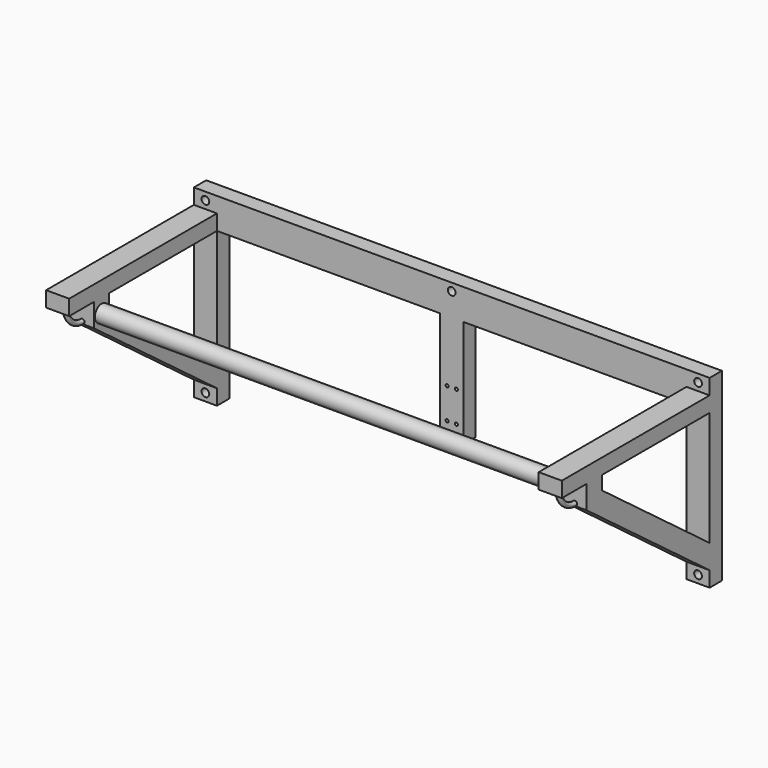
from build123d import *

# Parameters (mm, degrees)
F0_W           = 38.1
F0_H           = 25.4
F0_W_2         = 368.3
F0_H_2         = 177.8
F0_H_3         = 254
F1_DEPTH       = 25.4
F2_W           = 38.1
F2_H           = 25.4
F3_DEPTH       = 304.8
F4_W           = 850.9
F4_H           = 25.4
F5_DEPTH       = 25.4
F7_DEPTH       = 38.1
F9_DEPTH       = 38.1
F10_R          = 2.54
F11_DEPTH      = 12.7
F12_R          = 13.97
F13_DEPTH      = 406.4
F13_DEPTH_BACK = 406.4
F15_DEPTH      = 38.1
F17_DEPTH      = 38.1
F18_W          = 15.24
F18_H          = 39.0179467559
F19_DEPTH      = 50.8
F20_W          = 15.24
F20_H          = 39.0179467559
F21_DEPTH      = 50.8
F22_R          = 3.80999
F23_R          = 3.81
F24_DEPTH      = 25.4
F25_R          = 6.35
F26_DEPTH      = 12.7
F27_R          = 6.35
F28_DEPTH      = 12.7
F29_R          = 6.35
F30_DEPTH      = 12.7


# Not quite as in the source:
# - a fillet or chamfer is up to 0.001 mm smaller than in the source, because OpenCascade refuses the exact size


with BuildPart() as f1:
    # F0 (on Front) → F1 (new body)
    with BuildSketch(Plane.XZ):
        with Locations((0, 139.7)):
            Rectangle(F0_W, F0_H)
        with Locations((203.2, 114.3)):
            Rectangle(F0_W_2, F0_H)
        with Locations((0, 114.3)):
            Rectangle(F0_W, F0_H)
        with Locations((-203.2, 114.3)):
            Rectangle(F0_W_2, F0_H)
        with Locations((0, 12.7)):
            Rectangle(F0_W, F0_H_2)
        with Locations((406.4, 114.3)):
            Rectangle(F0_W, F0_H)
        with Locations((406.4, 139.7)):
            Rectangle(F0_W, F0_H)
        with Locations((-406.4, 139.7)):
            Rectangle(F0_W, F0_H)
        with Locations((-406.4, 114.3)):
            Rectangle(F0_W, F0_H)
        with Locations((406.4, -25.4)):
            Rectangle(F0_W, F0_H_3)
        with Locations((-406.4, -25.4)):
            Rectangle(F0_W, F0_H_3)
    extrude(amount=F1_DEPTH)

    # F2 (on face) → F3 (join)
    with BuildSketch(Plane.XZ.offset(25.4)):
        with Locations((-406.4, 114.3)):
            Rectangle(F2_W, F2_H)
        with Locations((406.4, 114.3)):
            Rectangle(F2_W, F2_H)
    extrude(amount=F3_DEPTH)

    # F4 (on face) → F5 (join)
    with BuildSketch(Plane.XZ.offset(25.4)):
        with Locations((0, 139.7)):
            Rectangle(F4_W, F4_H)
    extrude(amount=-F5_DEPTH)

    # F6 (on face) → F7 (join)
    with BuildSketch(Plane.YZ.offset(425.45)):
        Polygon((-279.4, 63.5), (-25.4, -127), (-25.4, -87.3125), (-247.65, 79.375), (-247.65, 101.6), (-279.4, 101.6), align=None)
    extrude(amount=-F7_DEPTH)

    # F8 (on face) → F9 (join)
    with BuildSketch(Plane.YZ.offset(-387.35)):
        Polygon((-279.4, 63.5), (-25.4, -127), (-25.4, -87.3125), (-247.65, 79.375), (-247.65, 101.6), (-279.4, 101.6), align=None)
    extrude(amount=-F9_DEPTH)

    # F10 (on face) → F11 (cut)
    with BuildSketch(Plane.XZ.offset(25.4)):
        with Locations((-7.62, 0)):
            Circle(F10_R)
        with Locations((7.62, 0)):
            Circle(F10_R)
        with Locations((-7.62, -50.8)):
            Circle(F10_R)
        with Locations((7.62, -50.8)):
            Circle(F10_R)
    extrude(amount=-F11_DEPTH, mode=Mode.SUBTRACT)

    # F12 (on Right) → F13 (join, two sides)
    with BuildSketch(Plane.YZ) as f13_sk:
        with Locations((-263.2673084736, 78.74)):
            Circle(F12_R)
    extrude(amount=-F13_DEPTH)
    extrude(f13_sk.sketch, amount=F13_DEPTH_BACK)

    # F14 (on face) → F15 (join)
    with BuildSketch(Plane(origin=(-425.45, 0, 0), x_dir=(0, -1, 0), z_dir=(-1, 0, 0))):
        with BuildLine():
            Line((279.4, 71.12), (279.4, 63.5))
            ThreePointArc((279.4, 63.5), (306.3407683632, 74.6592316368), (317.5, 101.6))
            Line((317.5, 101.6), (309.88, 101.6))
            ThreePointArc((309.88, 101.6), (300.9526146906, 80.0473853094), (279.4, 71.12))
        make_face()
    extrude(amount=-F15_DEPTH)

    # F16 (on face) → F17 (join)
    with BuildSketch(Plane(origin=(387.35, 0, 0), x_dir=(0, -1, 0), z_dir=(-1, 0, 0))):
        with BuildLine():
            Line((279.4, 71.12), (279.4, 63.5))
            ThreePointArc((279.4, 63.5), (306.3407683632, 74.6592316368), (317.5, 101.6))
            Line((317.5, 101.6), (309.88, 101.6))
            ThreePointArc((309.88, 101.6), (300.9526146906, 80.0473853094), (279.4, 71.12))
        make_face()
    extrude(amount=-F17_DEPTH)

    # F18 (on face) → F19 (cut)
    with BuildSketch(Plane.XZ.offset(330.2)):
        with Locations((-417.83, 82.0910266221)):
            Rectangle(F18_W, F18_H)
        with Locations((-394.97, 82.0910266221)):
            Rectangle(F18_W, F18_H)
    extrude(amount=-F19_DEPTH, mode=Mode.SUBTRACT)

    # F20 (on face) → F21 (cut)
    with BuildSketch(Plane.XZ.offset(330.2)):
        with Locations((394.97, 82.0910266221)):
            Rectangle(F20_W, F20_H)
        with Locations((417.83, 82.0910266221)):
            Rectangle(F20_W, F20_H)
    extrude(amount=-F21_DEPTH, mode=Mode.SUBTRACT)

    # F22 (radius 3.81 in the source; OpenCascade refuses exactly that, so slightly less here)
    f22_edges = [f1.edges().sort_by_distance(p)[0] for p in [
        (402.59, -306.340768, 74.659232),
        (402.59, -300.952615, 80.047385),
        (410.21, -306.340768, 74.659232),
        (410.21, -300.952615, 80.047385),
        (-410.21, -300.952615, 80.047385),
        (-410.21, -306.340768, 74.659232),
        (-402.59, -300.952615, 80.047385),
        (-402.59, -306.340768, 74.659232),
    ]]
    fillet(f22_edges, radius=F22_R)

    # F23 (on face) → F24 (cut)
    with BuildSketch(Plane(origin=(0, 0, 0), x_dir=(-1, 0, 0), z_dir=(0, 1, 0))):
        with Locations((0, 139.7)):
            Circle(F23_R)
        with Locations((-406.4, 139.7)):
            Circle(F23_R)
        with Locations((-406.4, -139.7)):
            Circle(F23_R)
        with Locations((406.4, -139.7)):
            Circle(F23_R)
        with Locations((406.4, 139.7)):
            Circle(F23_R)
    extrude(amount=-F24_DEPTH, mode=Mode.SUBTRACT)

    # F25 (on face) → F26 (cut)
    with BuildSketch(Plane.XZ.offset(25.4)):
        with Locations((-406.4, 139.7)):
            Circle(F25_R)
        with Locations((0, 139.7)):
            Circle(F25_R)
        with Locations((406.4, 139.7)):
            Circle(F25_R)
    extrude(amount=-F26_DEPTH, mode=Mode.SUBTRACT)

    # F27 (on face) → F28 (cut)
    with BuildSketch(Plane.XZ.offset(25.4)):
        with Locations((-406.4, -139.7)):
            Circle(F27_R)
    extrude(amount=-F28_DEPTH, mode=Mode.SUBTRACT)

    # F29 (on face) → F30 (cut)
    with BuildSketch(Plane.XZ.offset(25.4)):
        with Locations((406.4, -139.7)):
            Circle(F29_R)
    extrude(amount=-F30_DEPTH, mode=Mode.SUBTRACT)


solid = f1.part
